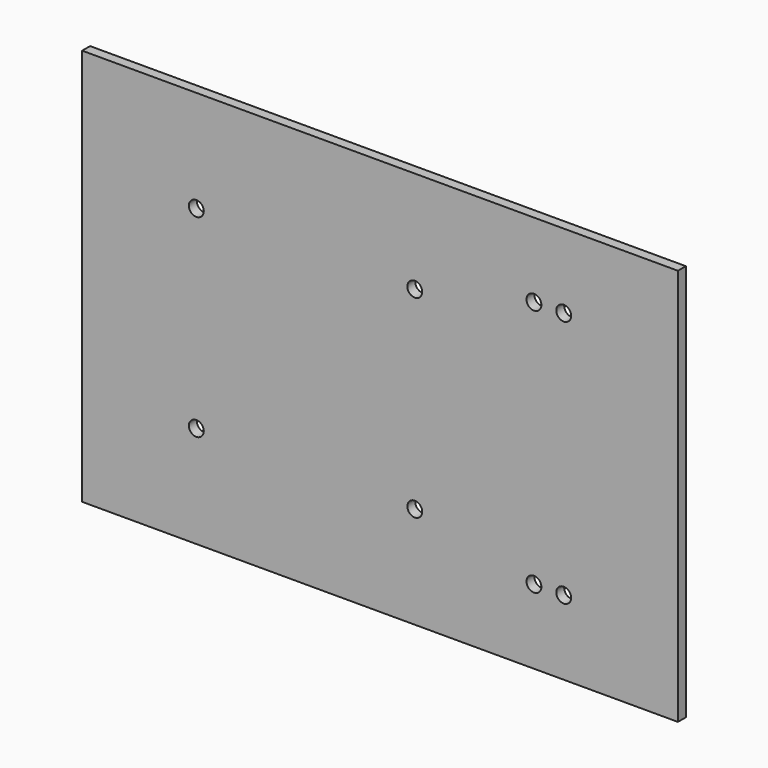
from build123d import *

# Parameters (mm, degrees)
F0_W     = 120
F0_H     = 80
F1_DEPTH = 2
F2_R     = 1.5
F3_DEPTH = 25


# Not quite as in the source:
# - a pattern or mirror of a feature is missing from the dataset's text; its kind, count and spacing are read off the source's solid


with BuildPart() as f1:
    # F0 (on Front) → F1 (new body)
    with BuildSketch(Plane.XZ):
        with Locations((60, 40)):
            Rectangle(F0_W, F0_H)
    extrude(amount=F1_DEPTH)

    # F2 (on face) → F3 (cut)
    with BuildSketch(Plane.XZ.offset(2)):
        with Locations((23, 59.5)):
            Circle(F2_R)
        with BuildLine():
            ThreePointArc((68.5, 59.5), (67, 61), (65.5, 59.5))
            ThreePointArc((65.5, 59.5), (67, 58), (68.5, 59.5))
        make_face()
        with Locations((91, 65)):
            Circle(F2_R)
        with BuildLine():
            ThreePointArc((98.5, 65), (97, 66.5), (95.5, 65))
            ThreePointArc((95.5, 65), (97, 63.5), (98.5, 65))
        make_face()
    f3 = extrude(amount=-F3_DEPTH, mode=Mode.SUBTRACT)

    # F3_copies: F3 across plane
    add(f3.mirror(Plane(origin=(0, 0, 40), x_dir=(-1, 0, 0), z_dir=(0, 0, -1))), mode=Mode.SUBTRACT)


solid = f1.part
